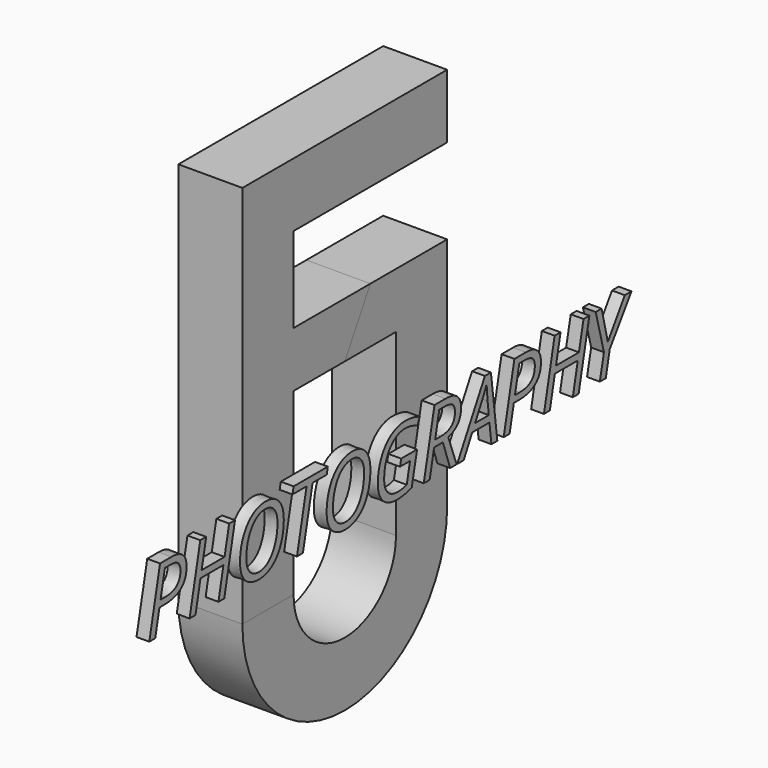
from build123d import *

# Parameters (mm, degrees)
F1_DEPTH     = 19.05
F2_DEPTH     = 19.05
F4_START     = 8.89
F3_TEXT_SIZE = 26.4583333333
F4_DEPTH     = 3.81


# Not quite as in the source:
# - Text() gives the source's letters only with a copy of the font that has no kerning and outlines rounded to 1/6400 em; it was checked with that copy


with BuildPart() as f1:
    # F0 (on Right) → F1 (new body)
    with BuildSketch(Plane.YZ):
        Polygon((-38.1, 114.3), (-38.1, 0), (-19.05, 0), (-19.05, 53.3522160579), (0, 53.3522160579), (9.525, 69.85), (-19.05, 69.85), (-19.05, 95.25), (38.1, 95.25), (38.1, 114.3), align=None)
    extrude(amount=-F1_DEPTH)


with BuildPart() as f2:
    # F0 (on Right) → F2 (new body)
    with BuildSketch(Plane.YZ):
        with BuildLine():
            Line((-19.05, 0), (-38.1, 0))
            ThreePointArc((-38.1, 0), (0, -38.1), (38.1, 0))
            Line((38.1, 0), (38.1, 69.85))
            Line((38.1, 69.85), (9.525, 69.85))
            Line((9.525, 69.85), (0, 53.3522160579))
            Line((0, 53.3522160579), (19.05, 53.3522160579))
            Line((19.05, 53.3522160579), (19.05, 0))
            ThreePointArc((19.05, 0), (0, -19.05), (-19.05, 0))
        make_face()
    extrude(amount=-F2_DEPTH)


with BuildPart() as f4:
    # F3 (on face) → F4 (new body)
    with BuildSketch(Plane.YZ.offset(F4_START)):
        with Locations((-89.7147813879, 20.0449441606)):
            Text('PHOTOGRAPHY', F3_TEXT_SIZE, font='Open Sans', font_style=FontStyle.ITALIC, text_align=(TextAlign.LEFT, TextAlign.BOTTOM))
    extrude(amount=F4_DEPTH)


solid = Compound([f1.part, f2.part, f4.part])
